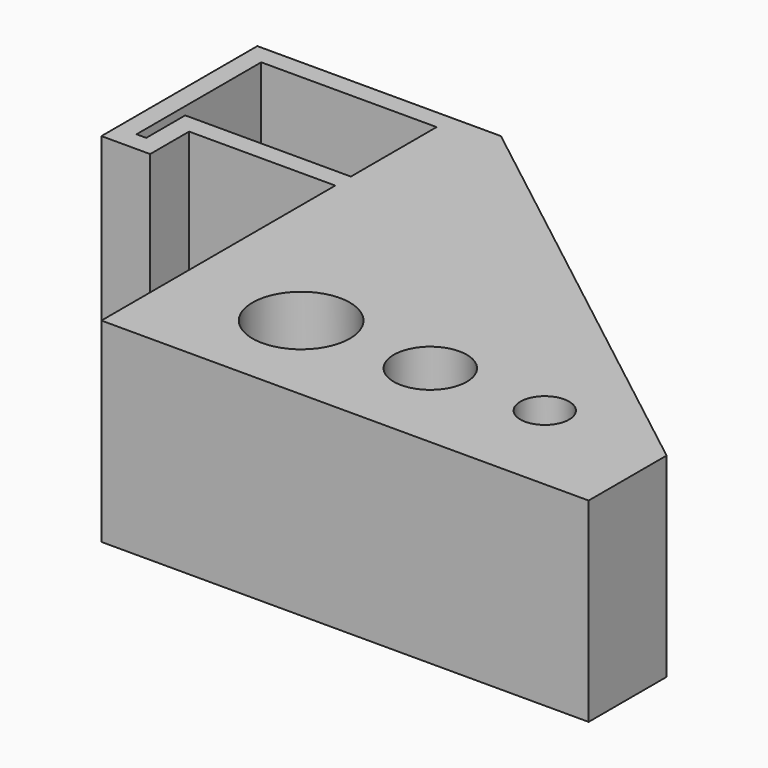
from build123d import *

# Parameters (mm, degrees)
F0_R     = 5
F0_R_2   = 3.75
F0_R_3   = 2.5
F1_DEPTH = 20
F2_DEPTH = 12.5
F4_DEPTH = 5
F5_DEPTH = 20.001


with BuildPart() as f1:
    # F0 (on Top) → F1 (new body)
    with BuildSketch(Plane.XY):
        Polygon((0, 7.4358002841), (0, -22.5641997159), (50, -22.5641997159), (50, -12.5641997159), (5, 22.4358002841), (-20, 22.4358002841), (-20, 2.4358002841), (-15, 2.4358002841), (-15, 7.4358002841), align=None)
        with Locations((12.5, -12.5641997159)):
            Circle(F0_R, mode=Mode.SUBTRACT)
        with Locations((25.75, -12.5641997159)):
            Circle(F0_R_2, mode=Mode.SUBTRACT)
        with Locations((37.5, -12.5641997159)):
            Circle(F0_R_3, mode=Mode.SUBTRACT)
        with Locations((12.5, -12.5641997159)):
            Circle(F0_R)
        with Locations((25.75, -12.5641997159)):
            Circle(F0_R_2)
        with Locations((37.5, -12.5641997159)):
            Circle(F0_R_3)
    extrude(amount=-F1_DEPTH)

    # F0 (on Top) → F2 (cut, symmetric)
    with BuildSketch(Plane.XY):
        with Locations((12.5, -12.5641997159)):
            Circle(F0_R)
        with Locations((25.75, -12.5641997159)):
            Circle(F0_R_2)
        with Locations((37.5, -12.5641997159)):
            Circle(F0_R_3)
    extrude(amount=F2_DEPTH, both=True, mode=Mode.SUBTRACT)

    # F3 (on face) → F4 (cut)
    with BuildSketch(Plane(origin=(0, 0, -20), x_dir=(1, 0, 0), z_dir=(0, 0, -1))):
        Polygon((20.7619503973, 0), (23.1309751987, 0), (24.3154875993, 2.0516356601), (23.1309751987, 2.7355142135), (22.0358983849, 2.1032713203), (21.9762746603, 2), (21.8570272111, 2), (20.7619503973, 1.3677571068), align=None)
        Polygon((20.7619503973, -1.3677571068), (20.7619503973, 0), (18.7619503973, 0), (18.7619503973, -2.5224576451), (23.1309751987, -5.0449152903), (27.5, -2.5224576451), (27.5, 2.5224576451), (25.3154875993, 3.7836864677), (24.3154875993, 2.0516356601), (25.5, 1.3677571068), (25.5, -1.3677571068), (23.1309751987, -2.7355142135), align=None)
        Polygon((18.7619503973, 0), (20.7619503973, 0), (20.7619503973, 1.3677571068), (21.8570272111, 2), (18.7619503973, 2), align=None)
        Polygon((23.1309751987, 2.7355142135), (24.3154875993, 2.0516356601), (25.3154875993, 3.7836864677), (23.5834367918, 4.7836864677), (22.0358983849, 2.1032713203), align=None)
        Polygon((14.3965897144, 0), (18.7619503973, 0), (18.7619503973, 2), (15.5512902527, 2), (12.338798049, 7.5641997159), (15.5512902527, 13.1283994317), (21.9762746603, 13.1283994317), (25.1887668641, 7.5641997159), (23.5834367918, 4.7836864677), (25.3154875993, 3.7836864677), (27.4981679408, 7.5641997159), (23.1309751987, 15.1283994317), (14.3965897144, 15.1283994317), (10.0293969722, 7.5641997159), align=None)
        Polygon((18.7619503973, 2.5224576451), (18.7619503973, 2), (21.8570272111, 2), (22.0358983849, 2.1032713203), (23.5834367918, 4.7836864677), (23.1309751987, 5.0449152903), align=None)
        Polygon((22.3340887545, 4.9830829416), (22.3218557052, 10.162153838), (17.3924863607, 11.7509404388), (14.358201612, 7.5537936626), (17.4122798502, 3.3710276983), align=None)
        Polygon((35.4952501059, 15.1283994317), (27.4952501059, 15.1283994317), (31.4952501059, 8.2001962014), align=None)
        Polygon((12.7505299598, -6.9282032303), (8.7505299598, 0), (4.7505299598, -6.9282032303), align=None)
        Polygon((0, -9.4358002841), (-15, -9.4358002841), (-17, -9.4358002841), (-17, -4.4358002841), (-18, -4.4358002841), (-18, -20.4358002841), (-15, -20.4358002841), (0, -20.4358002841), align=None)
    extrude(amount=-F4_DEPTH, mode=Mode.SUBTRACT)

    # F3 (on face) → F5 (cut, through all)
    with BuildSketch(Plane(origin=(0, 0, -20), x_dir=(1, 0, 0), z_dir=(0, 0, -1))):
        Polygon((0, -9.4358002841), (-15, -9.4358002841), (-17, -9.4358002841), (-17, -4.4358002841), (-18, -4.4358002841), (-18, -20.4358002841), (-15, -20.4358002841), (0, -20.4358002841), align=None)
    extrude(amount=-F5_DEPTH, mode=Mode.SUBTRACT)


solid = f1.part
